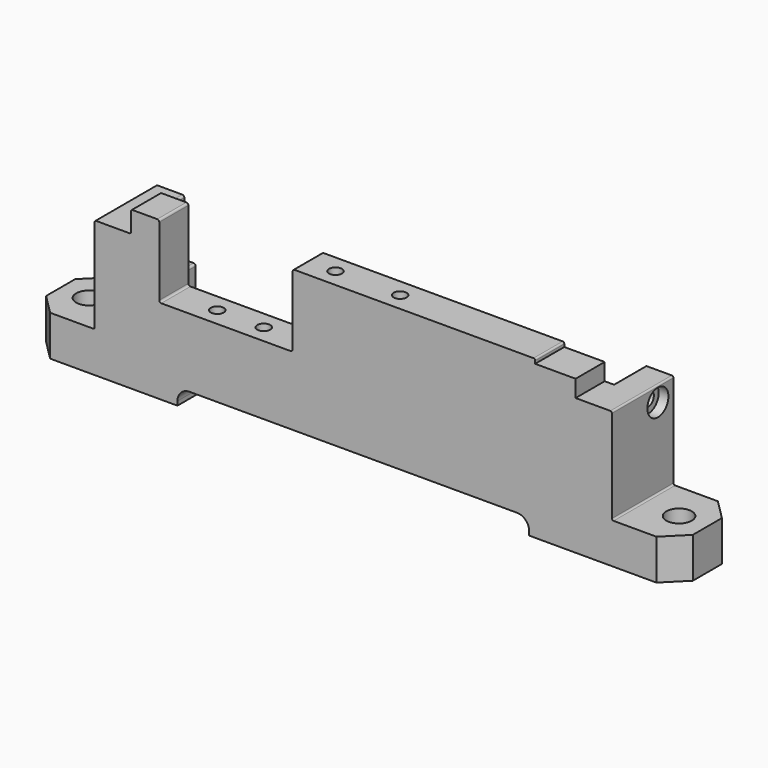
from build123d import *

# Parameters (mm, degrees)
F2_DEPTH  = 9
F3_DEPTH  = 10
F4_R      = 1.75
F5_DEPTH  = 158.2
F4_R_2    = 3.25
F6_DEPTH  = 2.4
F7_R      = 3.25
F8_DEPTH  = 2.4
F9_R      = 3.4
F9_R_2    = 1.75
F10_DEPTH = 3
F11_DEPTH = 25
F12_W     = 100
F12_H     = 9
F13_DEPTH = 1.1
F14_W     = 19
F14_H     = 10
F15_DEPTH = 16
F16_SIZE  = 5
F17_W     = 19
F17_H     = 10
F18_DEPTH = 16
F19_SIZE  = 5
F20_R     = 3.15
F21_DEPTH = 25
F22_R     = 0.4
F23_W     = 87
F23_H     = 9
F24_DEPTH = 4
F25_R     = 3
F26_W     = 33
F26_H     = 9
F26_R     = 1.6
F27_DEPTH = 18
F28_DEPTH = 30
F30_DEPTH = 2.6
F31_R     = 1.6
F32_DEPTH = 12.5
F34_DEPTH = 2.6
F35_W     = 5.5
F35_H     = 2.6
F36_DEPTH = 3.7
F37_R     = 0.5


with BuildPart() as f2:
    # F1 (on face) → F2 (new body)
    with BuildSketch(Plane.XZ):
        Polygon((-55, 27.7), (-64, 27.7), (-64, -6), (0, -6), (64, -6), (64, 27.7), (55, 27.7), (55, 31.9), (0, 31.9), (-55, 31.9), align=None)
    extrude(amount=F2_DEPTH)

    # F0 (on Front) → F3 (join)
    with BuildSketch(Plane.XZ):
        with BuildLine():
            Line((-57.5, 27.7), (-64, 27.7))
            Line((-64, 27.7), (-64, -6))
            Line((-64, -6), (-43.5, -6))
            Line((-43.5, -6), (-43.5, 0))
            Line((-43.5, 0), (-55, 0))
            ThreePointArc((-55, 0), (-55.3535533906, -0.1464466094), (-55.5, -0.5))
            Line((-55.5, -0.5), (-55.5, -1.8))
            Line((-55.5, -1.8), (-59, -1.8))
            Line((-59, -1.8), (-59, 6.2))
            Line((-59, 6.2), (-54.7, 6.2))
            ThreePointArc((-54.7, 6.2), (-54.3464466094, 6.3464466094), (-54.2, 6.7))
            Line((-54.2, 6.7), (-54.2, 13.2))
            ThreePointArc((-54.2, 13.2), (-54.3464466094, 13.5535533906), (-54.7, 13.7))
            Line((-54.7, 13.7), (-59, 13.7))
            Line((-59, 13.7), (-59, 20.2))
            Line((-59, 20.2), (-57.5, 20.2))
            ThreePointArc((-57.5, 20.2), (-57.1464466094, 20.3464466094), (-57, 20.7))
            Line((-57, 20.7), (-57, 27.2))
            ThreePointArc((-57, 27.2), (-57.1464466094, 27.5535533906), (-57.5, 27.7))
        make_face()
        with BuildLine():
            Line((43.5, -6), (64, -6))
            Line((64, -6), (64, 27.7))
            Line((64, 27.7), (57.5, 27.7))
            ThreePointArc((57.5, 27.7), (57.1464466094, 27.5535533906), (57, 27.2))
            Line((57, 27.2), (57, 20.7))
            ThreePointArc((57, 20.7), (57.1464466094, 20.3464466094), (57.5, 20.2))
            Line((57.5, 20.2), (59, 20.2))
            Line((59, 20.2), (59, 13.7))
            Line((59, 13.7), (54.7, 13.7))
            ThreePointArc((54.7, 13.7), (54.3464466094, 13.5535533906), (54.2, 13.2))
            Line((54.2, 13.2), (54.2, 6.7))
            ThreePointArc((54.2, 6.7), (54.3464466094, 6.3464466094), (54.7, 6.2))
            Line((54.7, 6.2), (59, 6.2))
            Line((59, 6.2), (59, -1.8))
            Line((59, -1.8), (55.5, -1.8))
            Line((55.5, -1.8), (55.5, -0.5))
            ThreePointArc((55.5, -0.5), (55.3535533906, -0.1464466094), (55, 0))
            Line((55, 0), (43.5, 0))
            Line((43.5, 0), (43.5, -6))
        make_face()
    extrude(amount=-F3_DEPTH)

    # F4 (on face) → F5 (cut)
    with BuildSketch(Plane(origin=(-64, 0, 0), x_dir=(0, -1, 0), z_dir=(-1, 0, 0))):
        with Locations((-5.2, 23.9)):
            Circle(F4_R)
    extrude(amount=-F5_DEPTH, mode=Mode.SUBTRACT)

    # F4 (on face) → F6 (cut)
    with BuildSketch(Plane(origin=(-64, 0, 0), x_dir=(0, -1, 0), z_dir=(-1, 0, 0))):
        with Locations((-5.2, 23.9)):
            Circle(F4_R_2)
        with Locations((-5.2, 23.9)):
            Circle(F4_R, mode=Mode.SUBTRACT)
    extrude(amount=-F6_DEPTH, mode=Mode.SUBTRACT)

    # F7 (on face) → F8 (cut)
    with BuildSketch(Plane.YZ.offset(64)):
        with Locations((5.2, 23.9)):
            Circle(F7_R)
    extrude(amount=-F8_DEPTH, mode=Mode.SUBTRACT)

    # F9 (on face) → F10 (cut)
    with BuildSketch(Plane(origin=(0, 0, -6), x_dir=(1, 0, 0), z_dir=(0, 0, -1))):
        with Locations((49.8, -5.1)):
            Circle(F9_R)
        with Locations((49.8, -5.1)):
            Circle(F9_R_2, mode=Mode.SUBTRACT)
        with Locations((-48.5, -5.1)):
            Circle(F9_R)
        with Locations((-48.5, -5.1)):
            Circle(F9_R_2, mode=Mode.SUBTRACT)
        with Locations((49.8, -5.1)):
            Circle(F9_R_2)
    extrude(amount=-F10_DEPTH, mode=Mode.SUBTRACT)

    # F9 (on face) → F11 (cut)
    with BuildSketch(Plane(origin=(0, 0, -6), x_dir=(1, 0, 0), z_dir=(0, 0, -1))):
        with Locations((49.8, -5.1)):
            Circle(F9_R_2)
        with Locations((-48.5, -5.1)):
            Circle(F9_R_2)
    extrude(amount=-F11_DEPTH, mode=Mode.SUBTRACT)

    # F12 (on face) → F13 (join)
    with BuildSketch(Plane.XY.offset(31.9)):
        with Locations((-5, -4.5)):
            Rectangle(F12_W, F12_H)
    extrude(amount=F13_DEPTH)

    # F14 (on face) → F15 (join)
    with BuildSketch(Plane(origin=(-64, 0, 0), x_dir=(0, -1, 0), z_dir=(-1, 0, 0))):
        with Locations((-0.5, -1)):
            Rectangle(F14_W, F14_H)
    extrude(amount=F15_DEPTH)

    # F16
    f16_edges = [f2.edges().sort_by_distance(p)[0] for p in [
        (-80, -9, -1),
        (-80, 10, -1),
    ]]
    chamfer(f16_edges, length=F16_SIZE)

    # F17 (on face) → F18 (join)
    with BuildSketch(Plane.YZ.offset(64)):
        with Locations((0.5, -1)):
            Rectangle(F17_W, F17_H)
    extrude(amount=F18_DEPTH)

    # F19
    f19_edges = [f2.edges().sort_by_distance(p)[0] for p in [
        (80, 10, -1),
        (80, -9, -1),
    ]]
    chamfer(f19_edges, length=F19_SIZE)

    # F20 (on face) → F21 (cut)
    with BuildSketch(Plane(origin=(0, 0, -6), x_dir=(1, 0, 0), z_dir=(0, 0, -1))):
        with Locations((-73, -0.5)):
            Circle(F20_R)
        with Locations((73, -0.5)):
            Circle(F20_R)
    extrude(amount=-F21_DEPTH, mode=Mode.SUBTRACT)

    # F22
    f22_edges = [f2.edges().sort_by_distance(p)[0] for p in [
        (64, 0.5, 27.7),
        (45, -4.5, 33),
        (-64, 0.5, 27.7),
        (-55, -4.5, 27.7),
        (-55, -4.5, 33),
        (-64, 0.5, 4),
        (64, 0.5, 4),
    ]]
    fillet(f22_edges, radius=F22_R)

    # F23 (on face) → F24 (cut)
    with BuildSketch(Plane(origin=(0, 0, -6), x_dir=(1, 0, 0), z_dir=(0, 0, -1))):
        with Locations((0, 4.5)):
            Rectangle(F23_W, F23_H)
    extrude(amount=-F24_DEPTH, mode=Mode.SUBTRACT)

    # F25
    f25_edges = [f2.edges().sort_by_distance(p)[0] for p in [
        (-43.5, -4.5, -2),
        (43.5, -4.5, -2),
    ]]
    fillet(f25_edges, radius=F25_R)

    # F26 (on face) → F27 (cut)
    with BuildSketch(Plane.XY.offset(33)):
        with Locations((-31.5, -4.5)):
            Rectangle(F26_W, F26_H)
        with Locations((-37.25, -4.5)):
            Circle(F26_R, mode=Mode.SUBTRACT)
        with Locations((-25.75, -4.5)):
            Circle(F26_R, mode=Mode.SUBTRACT)
    extrude(amount=-F27_DEPTH, mode=Mode.SUBTRACT)

    # F26 (on face) → F28 (cut)
    with BuildSketch(Plane.XY.offset(33)):
        with Locations((-37.25, -4.5)):
            Circle(F26_R)
        with Locations((-25.75, -4.5)):
            Circle(F26_R)
    extrude(amount=-F28_DEPTH, mode=Mode.SUBTRACT)

    # F29 (on face) → F30 (cut)
    with BuildSketch(Plane.XY.offset(3)):
        Polygon((-28.5, -2.9122867597), (-28.5, -6.0877132403), (-25.75, -7.6754264805), (-23, -6.0877132403), (-23, -2.9122867597), (-25.75, -1.3245735195), align=None)
        Polygon((-40, -2.9122867597), (-40, -6.0877132403), (-37.25, -7.6754264805), (-34.5, -6.0877132403), (-34.5, -2.9122867597), (-37.25, -1.3245735195), align=None)
    extrude(amount=F30_DEPTH, mode=Mode.SUBTRACT)

    # F31 (on face) → F32 (cut)
    with BuildSketch(Plane.XY.offset(33)):
        with Locations((-8, -4.5)):
            Circle(F31_R)
        with Locations((8, -4.5)):
            Circle(F31_R)
    extrude(amount=-F32_DEPTH, mode=Mode.SUBTRACT)

    # F33 (on face) → F34 (cut)
    with BuildSketch(Plane.XY.offset(20.5)):
        Polygon((-5.25, -6.0877132403), (-5.25, -2.9122867597), (-8, -1.3245735195), (-10.75, -2.9122867597), (-10.75, -6.0877132403), (-8, -7.6754264805), align=None)
        Polygon((10.75, -6.0877132403), (10.75, -2.9122867597), (8, -1.3245735195), (5.25, -2.9122867597), (5.25, -6.0877132403), (8, -7.6754264805), align=None)
    extrude(amount=F34_DEPTH, mode=Mode.SUBTRACT)

    # F35 (on face) → F36 (cut)
    with BuildSketch(Plane(origin=(0, 0, 0), x_dir=(-1, 0, 0), z_dir=(0, 1, 0))):
        with Locations((-8, 21.8)):
            Rectangle(F35_W, F35_H)
        with Locations((8, 21.8)):
            Rectangle(F35_W, F35_H)
        with Locations((25.75, 4.3)):
            Rectangle(F35_W, F35_H)
        with Locations((37.25, 4.3)):
            Rectangle(F35_W, F35_H)
    extrude(amount=-F36_DEPTH, mode=Mode.SUBTRACT)

    # F37
    f37_edges = [f2.edges().sort_by_distance(p)[0] for p in [
        (-15, -4.5, 33),
        (-15, -4.5, 15),
        (-48, -4.5, 15),
        (-48, -4.5, 33),
    ]]
    fillet(f37_edges, radius=F37_R)


solid = f2.part
